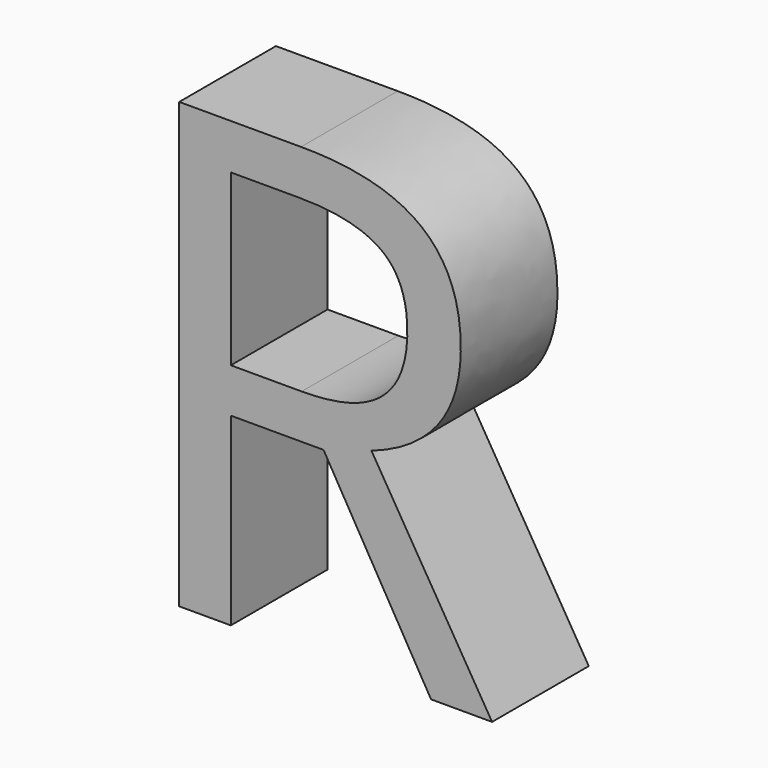
from build123d import *

# Parameters (mm, degrees)
F0_TEXT_SIZE = 51.4654805725
F1_DEPTH     = 10


# Not quite as in the source:
# - Text() gives the source's letters only with a copy of the font that has no kerning and outlines rounded to 1/6400 em; it was checked with that copy


with BuildPart() as f1:
    # F0 (on Front) → F1 (new body)
    with BuildSketch(Plane.XZ):
        with Locations((-34.2727934687, 0)):
            Text('R', F0_TEXT_SIZE, font='Open Sans', text_align=(TextAlign.LEFT, TextAlign.BOTTOM))
    extrude(amount=F1_DEPTH)


solid = f1.part
